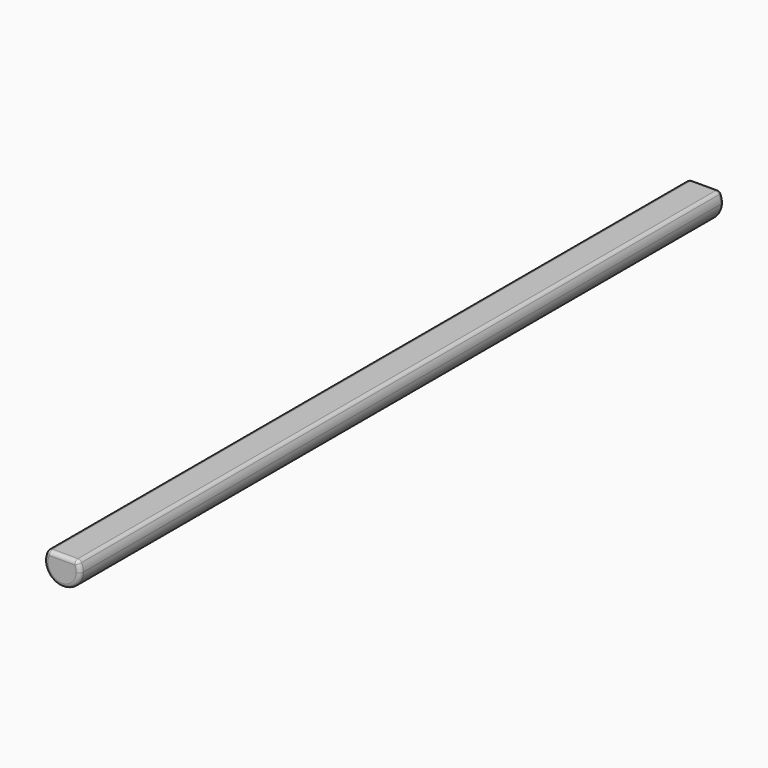
from build123d import *

# Parameters (mm, degrees)
F1_DEPTH = 101.6
F2_R     = 0.508


with BuildPart() as f1:
    # F0 (on Front) → F1 (new body)
    with BuildSketch(Plane.XZ):
        with BuildLine():
            ThreePointArc((-1.9007619525, 1.27), (-0.6635714644, -2.1875714644), (2.286, 0))
            ThreePointArc((2.286, 0), (2.1875714644, 0.6635714644), (1.9007619525, 1.27))
            Line((1.9007619525, 1.27), (-1.9007619525, 1.27))
        make_face()
    extrude(amount=F1_DEPTH)

    # F2
    f2_edges = [f1.edges().sort_by_distance(p)[0] for p in [
        (-1.900762, -50.8, 1.27),
        (0, -101.6, 1.27),
        (-0.663571, -101.6, -2.187571),
        (0, 0, 1.27),
        (-0.663571, 0, -2.187571),
        (1.900762, -50.8, 1.27),
    ]]
    fillet(f2_edges, radius=F2_R)


solid = f1.part
